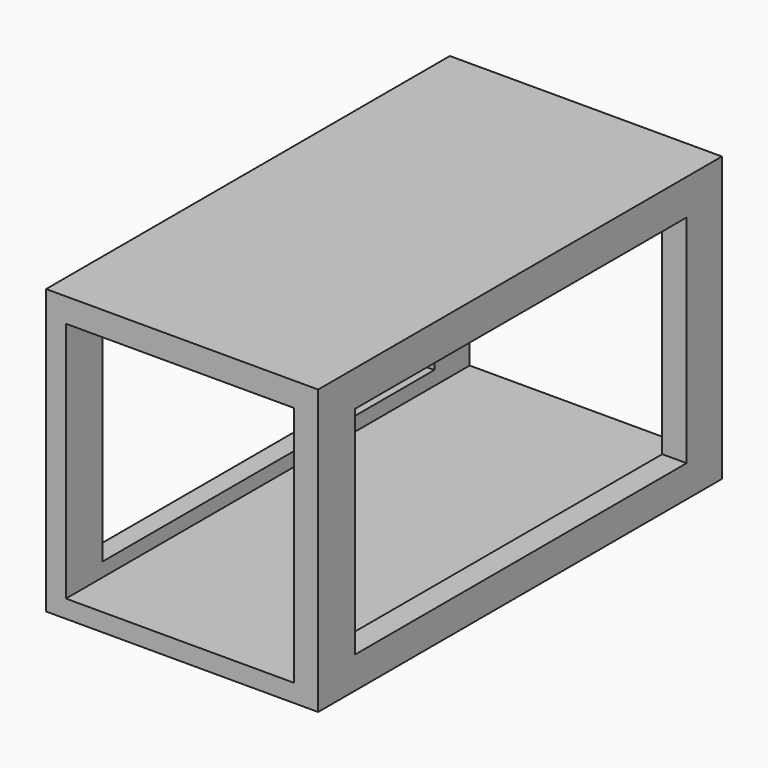
from build123d import *

# Parameters (mm, degrees)
F0_W         = 438.15
F0_H         = 457.2
F1_DEPTH     = 812.8
F2_TEXT_SIZE = 84.3270203414
F3_DEPTH     = 25.4
F4_W         = 366.9508397579
F4_H         = 389.6552473307
F5_DEPTH     = 812.801
F6_W         = 667.8473204374
F6_H         = 348.393894732
F7_DEPTH     = 438.151


# Not quite as in the source:
# - Text() gives the source's letters only with a copy of the font that has no kerning and outlines rounded to 1/6400 em; it was checked with that copy


with BuildPart() as f1:
    # F0 (on Front) → F1 (new body)
    with BuildSketch(Plane.XZ):
        Rectangle(F0_W, F0_H)
    extrude(amount=-F1_DEPTH)

    # F2 (on face) → F3 (cut)
    with BuildSketch(Plane.XZ):
        with Locations((-62.6918691851, -36.5901999176)):
            Text('TIG', F2_TEXT_SIZE, font='Open Sans', text_align=(TextAlign.LEFT, TextAlign.BOTTOM))
    extrude(amount=-F3_DEPTH, mode=Mode.SUBTRACT)

    # F4 (on face) → F5 (cut, through all)
    with BuildSketch(Plane.XZ):
        with Locations((-3.6268383265, -5.0259307027)):
            Rectangle(F4_W, F4_H)
    extrude(amount=-F5_DEPTH, mode=Mode.SUBTRACT)

    # F6 (on face) → F7 (cut, through all)
    with BuildSketch(Plane.YZ.offset(219.075)):
        with Locations((407.7475816011, -3.1201206148)):
            Rectangle(F6_W, F6_H)
    extrude(amount=-F7_DEPTH, mode=Mode.SUBTRACT)


solid = f1.part
